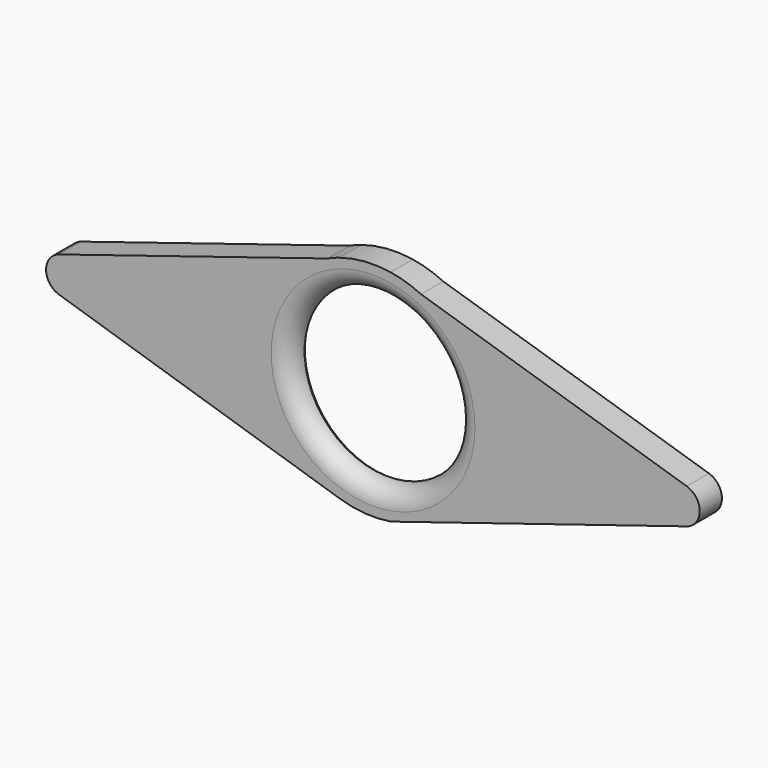
from build123d import *

# Parameters (mm, degrees)
F0_R     = 11.43
F1_DEPTH = 3.81
F2_R     = 2.54


# Not quite as in the source:
# - a fillet or chamfer that OpenCascade refuses, or shapes differently, is made with other operations: its cross-section is extruded or revolved along the edge and cut away or added


with BuildPart() as f1:
    # F0 (on Front) → F1 (new body)
    with BuildSketch(Plane.XZ):
        with BuildLine():
            Line((6.5569237481, 13.7573380769), (2.4006070358, 15.0497403918))
            ThreePointArc((2.4006070358, 15.0497403918), (-1.1592691439, 15.195844664), (-4.6557853401, 14.5114183617))
            ThreePointArc((-4.6557853401, 14.5114183617), (-5.4590945375, 14.2286994076), (-6.2453574463, 13.9015506462))
            Line((-6.2453574463, 13.9015506462), (-50.8, 0))
            Line((-50.8, 0), (-4.5719998884, -14.5380334647))
            ThreePointArc((-4.5719998884, -14.5380334647), (-1.1154361142, -15.1991250497), (2.4006070358, -15.0497403918))
            Line((2.4006070358, -15.0497403918), (50.8, 0))
            Line((50.8, 0), (6.5569237481, 13.7573380769))
        make_face()
        Circle(F0_R, mode=Mode.SUBTRACT)
        with BuildLine():
            ThreePointArc((6.5569237481, 13.7573380769), (4.5251425803, 14.552686509), (2.4006070358, 15.0497403918))
            Line((2.4006070358, 15.0497403918), (6.5569237481, 13.7573380769))
        make_face()
    extrude(amount=F1_DEPTH)

    # F2
    f2_edges = [f1.edges().sort_by_distance(p)[0] for p in [
        (50.8, -1.905, 0),
        (-50.8, -1.905, 0),
        (-11.43, -3.81, 0),
    ]]
    fillet(f2_edges, radius=F2_R)

    # F3: fillet of radius 2.54 on 1 edges, made by hand

    # F3_s1 → F3_t2 (revolve, cut)
    with BuildSketch(Plane.XY):
        with BuildLine():
            ThreePointArc((13.6297045256, 0), (12.3597045256, -0.3402954744), (11.43, -1.27))
            Line((11.43, -1.27), (11.43, 0))
            Line((11.43, 0), (13.6297045256, 0))
        make_face()
    revolve(axis=Axis((0, 0, 0), (0, -1, 0)), mode=Mode.SUBTRACT)


solid = f1.part
